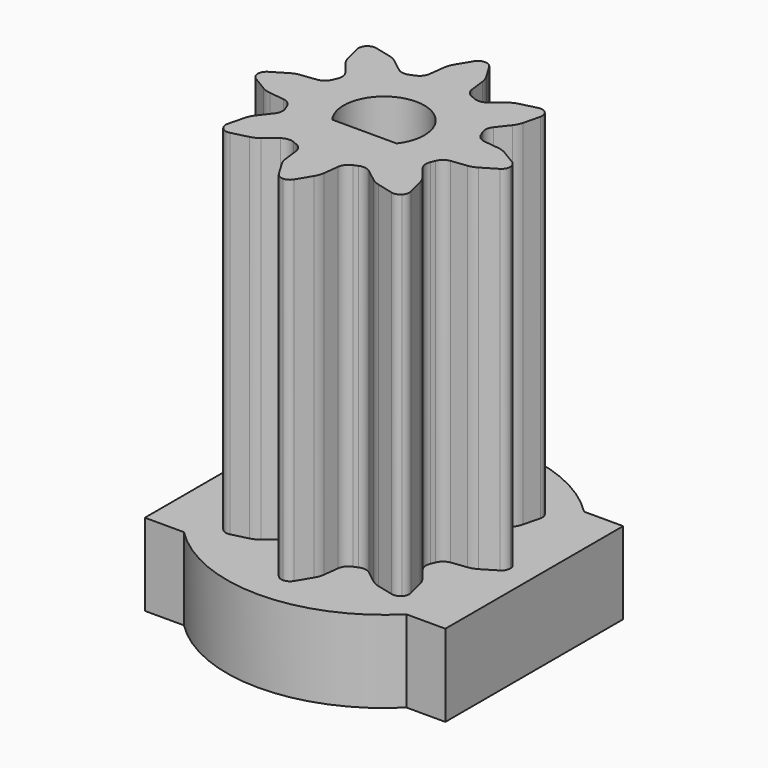
from build123d import *

# Parameters (mm, degrees)
F0_R     = 5
F0_R_2   = 3.15
F0_R_3   = 2.55
F1_DEPTH = 3.25
F2_R     = 2.55
F3_DEPTH = 14


# Not quite as in the source:
# - a feature names something its author has since deleted; it is built from what else it names


with BuildPart() as f1:
    # F0 (on Top) → F1 (new body)
    with BuildSketch(Plane.XY):
        with BuildLine():
            Line((-5.95, -4.4), (-4.4034787385, -4.4))
            ThreePointArc((-4.4034787385, -4.4), (0, -6.225), (4.4034787385, -4.4))
            Line((4.4034787385, -4.4), (5.95, -4.4))
            Line((5.95, -4.4), (5.95, 4.4))
            Line((5.95, 4.4), (4.4034787385, 4.4))
            ThreePointArc((4.4034787385, 4.4), (0, 6.225), (-4.4034787385, 4.4))
            Line((-4.4034787385, 4.4), (-5.95, 4.4))
            Line((-5.95, 4.4), (-5.95, -4.4))
        make_face()
        Circle(F0_R, mode=Mode.SUBTRACT)
        Circle(F0_R)
        Circle(F0_R_2, mode=Mode.SUBTRACT)
        Circle(F0_R_2)
        Circle(F0_R_3, mode=Mode.SUBTRACT)
        Circle(F0_R_3)
        with BuildLine():
            ThreePointArc((-1.275, -0.9666307465), (-0.5099019514, 1.5165750888), (1.6, 0))
            ThreePointArc((1.6, 0), (1.5165750888, -0.5099019514), (1.275, -0.9666307465))
            ThreePointArc((1.275, -0.9666307465), (0, -1.6), (-1.275, -0.9666307465))
        make_face(mode=Mode.SUBTRACT)
        with BuildLine():
            Line((1.275, -0.9666307465), (-1.275, -0.9666307465))
            ThreePointArc((-1.275, -0.9666307465), (0, -1.6), (1.275, -0.9666307465))
        make_face()
    extrude(amount=F1_DEPTH)

    # F2 (on face) → F3 (join)
    with BuildSketch(Plane.XY.offset(3.25)):
        with BuildLine():
            ThreePointArc((-4.8302633262, 0.3000085552), (-4.9546244936, 0.172348246), (-5, 0))
            ThreePointArc((-5, 0), (-4.9546244936, -0.172348246), (-4.8302633262, -0.3000085552))
            Line((-4.8302633262, -0.3000085552), (-4.2601369618, -0.6425750355))
            ThreePointArc((-4.2601369618, -0.6425750355), (-4.0929165173, -0.7205512094), (-3.9131380826, -0.7620563314))
            Line((-3.9131380826, -0.7620563314), (-3.3117988826, -0.835891501))
            ThreePointArc((-3.3117988826, -0.835891501), (-3.0868883315, -0.9291389359), (-2.9422567869, -1.125))
            ThreePointArc((-2.9422567869, -1.125), (-3.15, 0), (-2.9422567869, 1.125))
            ThreePointArc((-2.9422567869, 1.125), (-3.0868883315, 0.9291389359), (-3.3117988826, 0.835891501))
            Line((-3.3117988826, 0.835891501), (-3.9131380826, 0.7620563314))
            ThreePointArc((-3.9131380826, 0.7620563314), (-4.0929165173, 0.7205512094), (-4.2601369618, 0.6425750355))
            Line((-4.2601369618, 0.6425750355), (-4.8302633262, 0.3000085552))
        make_face()
        with BuildLine():
            ThreePointArc((-3.2033738691, 3.6276500367), (-3.3815799641, 3.6253171911), (-3.5355339059, 3.5355339059))
            ThreePointArc((-3.5355339059, 3.5355339059), (-3.6253171911, 3.3815799641), (-3.6276500367, 3.2033738691))
            Line((-3.6276500367, 3.2033738691), (-3.4667408995, 2.5580025694))
            ThreePointArc((-3.4667408995, 2.5580025694), (-3.4036356706, 2.3846223779), (-3.3058616735, 2.2281512744))
            Line((-3.3058616735, 2.2281512744), (-2.9328599965, 1.7507308991))
            ThreePointArc((-2.9328599965, 1.7507308991), (-2.8397601142, 1.5257592297), (-2.8759848548, 1.2849945972))
            ThreePointArc((-2.8759848548, 1.2849945972), (-2.2273863607, 2.2273863607), (-1.2849945972, 2.8759848548))
            ThreePointArc((-1.2849945972, 2.8759848548), (-1.5257592297, 2.8397601142), (-1.7507308991, 2.9328599965))
            Line((-1.7507308991, 2.9328599965), (-2.2281512744, 3.3058616735))
            ThreePointArc((-2.2281512744, 3.3058616735), (-2.3846223779, 3.4036356706), (-2.5580025694, 3.4667408995))
            Line((-2.5580025694, 3.4667408995), (-3.2033738691, 3.6276500367))
        make_face()
        with BuildLine():
            ThreePointArc((0.3000085552, 4.8302633262), (0.172348246, 4.9546244936), (0, 5))
            ThreePointArc((0, 5), (-0.172348246, 4.9546244936), (-0.3000085552, 4.8302633262))
            Line((-0.3000085552, 4.8302633262), (-0.6425750355, 4.2601369618))
            ThreePointArc((-0.6425750355, 4.2601369618), (-0.7205512094, 4.0929165173), (-0.7620563314, 3.9131380826))
            Line((-0.7620563314, 3.9131380826), (-0.835891501, 3.3117988826))
            ThreePointArc((-0.835891501, 3.3117988826), (-0.9291389359, 3.0868883315), (-1.125, 2.9422567869))
            ThreePointArc((-1.125, 2.9422567869), (0, 3.15), (1.125, 2.9422567869))
            ThreePointArc((1.125, 2.9422567869), (0.9291389359, 3.0868883315), (0.835891501, 3.3117988826))
            Line((0.835891501, 3.3117988826), (0.7620563314, 3.9131380826))
            ThreePointArc((0.7620563314, 3.9131380826), (0.7205512094, 4.0929165173), (0.6425750355, 4.2601369618))
            Line((0.6425750355, 4.2601369618), (0.3000085552, 4.8302633262))
        make_face()
        with BuildLine():
            ThreePointArc((3.2033738691, -3.6276500367), (3.3815799667, -3.6253171904), (3.5355339096, -3.5355339023))
            ThreePointArc((3.5355339096, -3.5355339023), (3.6253171918, -3.3815799616), (3.6276500367, -3.2033738691))
            Line((3.6276500367, -3.2033738691), (3.4667408995, -2.5580025694))
            ThreePointArc((3.4667408995, -2.5580025694), (3.4036356706, -2.3846223779), (3.3058616735, -2.2281512744))
            Line((3.3058616735, -2.2281512744), (2.9328599965, -1.7507308991))
            ThreePointArc((2.9328599965, -1.7507308991), (2.8397601142, -1.5257592297), (2.8759848548, -1.2849945972))
            ThreePointArc((2.8759848548, -1.2849945972), (2.2273863607, -2.2273863607), (1.2849945972, -2.8759848548))
            ThreePointArc((1.2849945972, -2.8759848548), (1.5257592297, -2.8397601142), (1.7507308991, -2.9328599965))
            Line((1.7507308991, -2.9328599965), (2.2281512744, -3.3058616735))
            ThreePointArc((2.2281512744, -3.3058616735), (2.3846223779, -3.4036356706), (2.5580025694, -3.4667408995))
            Line((2.5580025694, -3.4667408995), (3.2033738691, -3.6276500367))
        make_face()
        with BuildLine():
            ThreePointArc((-0.3000085552, -4.8302633262), (-0.172348246, -4.9546244936), (0, -5))
            ThreePointArc((0, -5), (0.172348246, -4.9546244936), (0.3000085552, -4.8302633262))
            Line((0.3000085552, -4.8302633262), (0.6425750355, -4.2601369618))
            ThreePointArc((0.6425750355, -4.2601369618), (0.7205512094, -4.0929165173), (0.7620563314, -3.9131380826))
            Line((0.7620563314, -3.9131380826), (0.835891501, -3.3117988826))
            ThreePointArc((0.835891501, -3.3117988826), (0.9291389359, -3.0868883315), (1.125, -2.9422567869))
            ThreePointArc((1.125, -2.9422567869), (0, -3.15), (-1.125, -2.9422567869))
            ThreePointArc((-1.125, -2.9422567869), (-0.9291389359, -3.0868883315), (-0.835891501, -3.3117988826))
            Line((-0.835891501, -3.3117988826), (-0.7620563314, -3.9131380826))
            ThreePointArc((-0.7620563314, -3.9131380826), (-0.7205512094, -4.0929165173), (-0.6425750355, -4.2601369618))
            Line((-0.6425750355, -4.2601369618), (-0.3000085552, -4.8302633262))
        make_face()
        with BuildLine():
            ThreePointArc((-3.6276500367, -3.2033738691), (-3.6253171911, -3.3815799641), (-3.5355339059, -3.5355339059))
            ThreePointArc((-3.5355339059, -3.5355339059), (-3.3815799641, -3.6253171911), (-3.2033738691, -3.6276500367))
            Line((-3.2033738691, -3.6276500367), (-2.5580025694, -3.4667408995))
            ThreePointArc((-2.5580025694, -3.4667408995), (-2.3846223779, -3.4036356706), (-2.2281512744, -3.3058616735))
            Line((-2.2281512744, -3.3058616735), (-1.7507308991, -2.9328599965))
            ThreePointArc((-1.7507308991, -2.9328599965), (-1.5257592297, -2.8397601142), (-1.2849945972, -2.8759848548))
            ThreePointArc((-1.2849945972, -2.8759848548), (-2.2273863607, -2.2273863607), (-2.8759848548, -1.2849945972))
            ThreePointArc((-2.8759848548, -1.2849945972), (-2.8397601142, -1.5257592297), (-2.9328599965, -1.7507308991))
            Line((-2.9328599965, -1.7507308991), (-3.3058616735, -2.2281512744))
            ThreePointArc((-3.3058616735, -2.2281512744), (-3.4036356706, -2.3846223779), (-3.4667408995, -2.5580025694))
            Line((-3.4667408995, -2.5580025694), (-3.6276500367, -3.2033738691))
        make_face()
        with BuildLine():
            ThreePointArc((2.8759848548, -1.2849945972), (2.9102205274, -1.205452812), (2.9422567869, -1.125))
            ThreePointArc((2.9422567869, -1.125), (3.0976288414, -0.5720101054), (3.15, 0))
            ThreePointArc((3.15, 0), (3.0976288414, 0.5720101054), (2.9422567869, 1.125))
            ThreePointArc((2.9422567869, 1.125), (2.9102205274, 1.205452812), (2.8759848548, 1.2849945972))
            ThreePointArc((2.8759848548, 1.2849945972), (2.2273863607, 2.2273863607), (1.2849945972, 2.8759848548))
            ThreePointArc((1.2849945972, 2.8759848548), (1.205452812, 2.9102205274), (1.125, 2.9422567869))
            ThreePointArc((1.125, 2.9422567869), (0, 3.15), (-1.125, 2.9422567869))
            ThreePointArc((-1.125, 2.9422567869), (-1.205452812, 2.9102205274), (-1.2849945972, 2.8759848548))
            ThreePointArc((-1.2849945972, 2.8759848548), (-2.2273863607, 2.2273863607), (-2.8759848548, 1.2849945972))
            ThreePointArc((-2.8759848548, 1.2849945972), (-2.9102205274, 1.205452812), (-2.9422567869, 1.125))
            ThreePointArc((-2.9422567869, 1.125), (-3.15, 0), (-2.9422567869, -1.125))
            ThreePointArc((-2.9422567869, -1.125), (-2.9102205274, -1.205452812), (-2.8759848548, -1.2849945972))
            ThreePointArc((-2.8759848548, -1.2849945972), (-2.2273863607, -2.2273863607), (-1.2849945972, -2.8759848548))
            ThreePointArc((-1.2849945972, -2.8759848548), (-1.205452812, -2.9102205274), (-1.125, -2.9422567869))
            ThreePointArc((-1.125, -2.9422567869), (0, -3.15), (1.125, -2.9422567869))
            ThreePointArc((1.125, -2.9422567869), (1.205452812, -2.9102205274), (1.2849945972, -2.8759848548))
            ThreePointArc((1.2849945972, -2.8759848548), (2.2273863607, -2.2273863607), (2.8759848548, -1.2849945972))
        make_face()
        Circle(F2_R, mode=Mode.SUBTRACT)
        Circle(F2_R)
        with BuildLine():
            ThreePointArc((-1.275, -0.9666307465), (0, 1.6), (1.275, -0.9666307465))
            Line((1.275, -0.9666307465), (-1.275, -0.9666307465))
        make_face(mode=Mode.SUBTRACT)
        with BuildLine():
            ThreePointArc((3.6276500367, 3.2033738691), (3.6253171915, 3.3815799629), (3.5355339078, 3.5355339041))
            ThreePointArc((3.5355339078, 3.5355339041), (3.3815799654, 3.6253171908), (3.2033738691, 3.6276500367))
            Line((3.2033738691, 3.6276500367), (2.5580025694, 3.4667408995))
            ThreePointArc((2.5580025694, 3.4667408995), (2.3846223779, 3.4036356706), (2.2281512744, 3.3058616735))
            Line((2.2281512744, 3.3058616735), (1.7507308991, 2.9328599965))
            ThreePointArc((1.7507308991, 2.9328599965), (1.5257592297, 2.8397601142), (1.2849945972, 2.8759848548))
            ThreePointArc((1.2849945972, 2.8759848548), (2.2273863607, 2.2273863607), (2.8759848548, 1.2849945972))
            ThreePointArc((2.8759848548, 1.2849945972), (2.8397601142, 1.5257592297), (2.9328599965, 1.7507308991))
            Line((2.9328599965, 1.7507308991), (3.3058616735, 2.2281512744))
            ThreePointArc((3.3058616735, 2.2281512744), (3.4036356706, 2.3846223779), (3.4667408995, 2.5580025694))
            Line((3.4667408995, 2.5580025694), (3.6276500367, 3.2033738691))
        make_face()
        with BuildLine():
            ThreePointArc((4.8302633262, -0.3000085552), (4.9546244936, -0.172348246), (5, 0))
            ThreePointArc((5, 0), (4.9546244936, 0.172348246), (4.8302633262, 0.3000085552))
            Line((4.8302633262, 0.3000085552), (4.2601369618, 0.6425750355))
            ThreePointArc((4.2601369618, 0.6425750355), (4.0929165173, 0.7205512094), (3.9131380826, 0.7620563314))
            Line((3.9131380826, 0.7620563314), (3.3117988826, 0.835891501))
            ThreePointArc((3.3117988826, 0.835891501), (3.0868883315, 0.9291389359), (2.9422567869, 1.125))
            ThreePointArc((2.9422567869, 1.125), (3.0976288414, 0.5720101054), (3.15, 0))
            ThreePointArc((3.15, 0), (3.0976288414, -0.5720101054), (2.9422567869, -1.125))
            ThreePointArc((2.9422567869, -1.125), (3.0868883315, -0.9291389359), (3.3117988826, -0.835891501))
            Line((3.3117988826, -0.835891501), (3.9131380826, -0.7620563314))
            ThreePointArc((3.9131380826, -0.7620563314), (4.0929165173, -0.7205512094), (4.2601369618, -0.6425750355))
            Line((4.2601369618, -0.6425750355), (4.8302633262, -0.3000085552))
        make_face()
    extrude(amount=F3_DEPTH)


solid = f1.part
